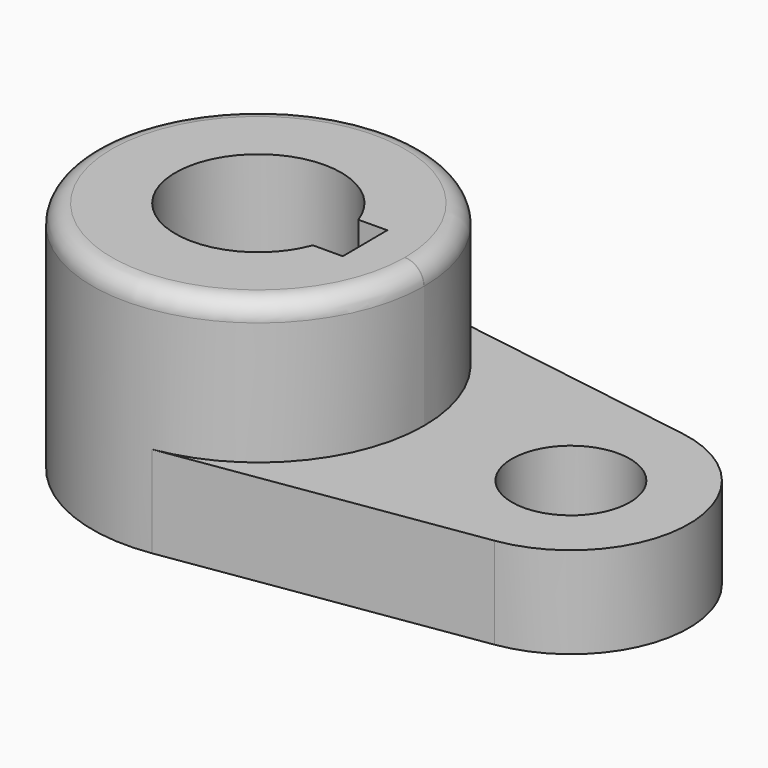
from build123d import *

# Parameters (mm, degrees)
F1_DEPTH = 15.7734
F2_DEPTH = 40.2336
F3_R     = 3.302


# Not quite as in the source:
# - a feature names something its author has since deleted; it is built from what else it names


with BuildPart() as f1:
    # F0 (on Top) → F1 (new body)
    with BuildSketch(Plane.XY):
        with BuildLine():
            ThreePointArc((28.5749057346, -0.0733979643), (28.5749764336, -0.0366990124), (28.575, 0))
            ThreePointArc((28.575, 0), (21.7196871584, 18.5684090525), (4.4430094671, 28.2274740612))
            ThreePointArc((4.4430094671, 28.2274740612), (-28.5749057039, 0.0734099128), (4.2979170796, -28.2499298013))
            ThreePointArc((4.2979170796, -28.2499298013), (21.6479758068, -18.6519641987), (28.5749057346, -0.0733979643))
        make_face()
        with BuildLine():
            Line((18.4686649637, 4.6872641706), (18.4984100104, -0.0475153147))
            Line((18.4984100104, -0.0475153147), (18.5293, -4.9645453691))
            Line((18.5293, -4.9645453691), (13.3852167998, -4.9968617623))
            ThreePointArc((13.3852167998, -4.9968617623), (-14.2863531341, 0.1810259026), (13.5075318215, 4.6560971147))
            Line((13.5075318215, 4.6560971147), (18.4686649637, 4.6872641706))
        make_face(mode=Mode.SUBTRACT)
        with BuildLine():
            ThreePointArc((4.4430094671, 28.2274740612), (21.7196871584, 18.5684090525), (28.575, 0))
            ThreePointArc((28.575, 0), (28.5749764336, -0.0366990124), (28.5749057346, -0.0733979643))
            ThreePointArc((28.5749057346, -0.0733979643), (21.6479758068, -18.6519641987), (4.2979170796, -28.2499298013))
            Line((4.2979170796, -28.2499298013), (56.9175468923, -20.2444300608))
            ThreePointArc((56.9175468923, -20.2444300608), (74.2947643422, -0.1870234197), (57.0132588055, 19.9529074106))
            Line((57.0132588055, 19.9529074106), (4.4430094671, 28.2274740612))
        make_face()
        with BuildLine():
            ThreePointArc((64.1348219431, -0.1386405993), (53.9617734053, -10.2986322201), (43.8148554597, -0.1125435453))
            ThreePointArc((43.8148554597, -0.1125435453), (53.9878704808, 10.0213510216), (64.1348219431, -0.1386405993))
        make_face(mode=Mode.SUBTRACT)
    extrude(amount=F1_DEPTH)

    # F0 (on Top) → F2 (join)
    with BuildSketch(Plane.XY):
        with BuildLine():
            ThreePointArc((28.5749057346, -0.0733979643), (28.5749764336, -0.0366990124), (28.575, 0))
            ThreePointArc((28.575, 0), (21.7196871584, 18.5684090525), (4.4430094671, 28.2274740612))
            ThreePointArc((4.4430094671, 28.2274740612), (-28.5749057039, 0.0734099128), (4.2979170796, -28.2499298013))
            ThreePointArc((4.2979170796, -28.2499298013), (21.6479758068, -18.6519641987), (28.5749057346, -0.0733979643))
        make_face()
        with BuildLine():
            Line((18.4686649637, 4.6872641706), (18.4984100104, -0.0475153147))
            Line((18.4984100104, -0.0475153147), (18.5293, -4.9645453691))
            Line((18.5293, -4.9645453691), (13.3852167998, -4.9968617623))
            ThreePointArc((13.3852167998, -4.9968617623), (-14.2863531341, 0.1810259026), (13.5075318215, 4.6560971147))
            Line((13.5075318215, 4.6560971147), (18.4686649637, 4.6872641706))
        make_face(mode=Mode.SUBTRACT)
    extrude(amount=F2_DEPTH)

    # F3
    f3_edges = [f1.edges().sort_by_distance(p)[0] for p in [
        (-4.297917, 28.24993, 40.2336),
    ]]
    fillet(f3_edges, radius=F3_R)


solid = f1.part
